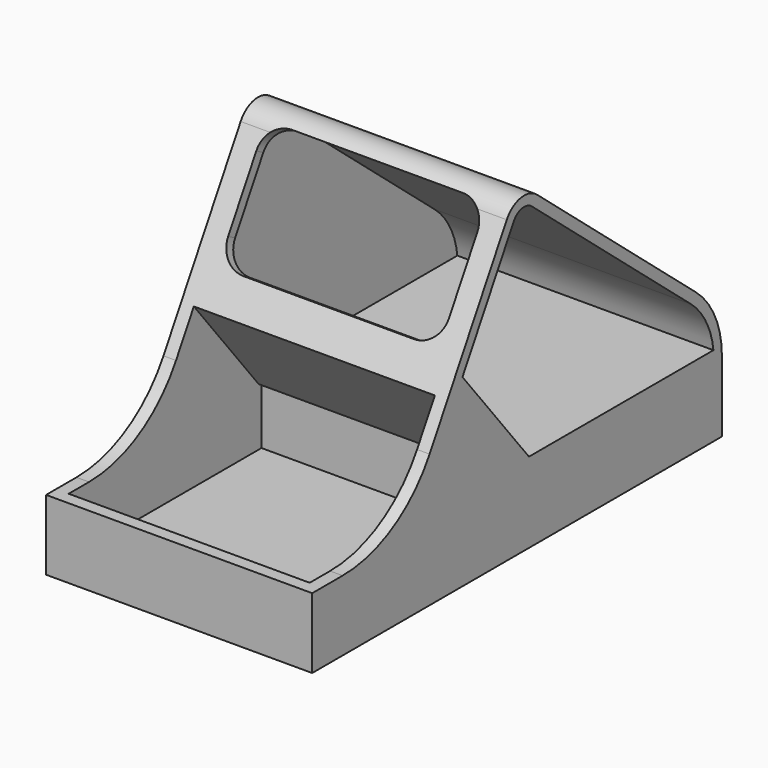
from build123d import *

# Parameters (mm, degrees)
F0_W      = 53
F0_H      = 53
F1_DEPTH  = 14
F0_H_2    = 49
F2_DEPTH  = 14
F3_T      = -2.5
F5_DEPTH  = 53
F6_DEPTH  = 53
F7_T      = -2.5
F9_R      = 18
F10_R     = 5
F11_T     = -2
F12_DEPTH = 7.2
F14_R     = 25


with BuildPart() as f1:
    # F0 (on Top) → F1 (new body)
    with BuildSketch(Plane.XY):
        with Locations((0, -24.5)):
            Rectangle(F0_W, F0_H)
    extrude(amount=F1_DEPTH)

    # F3
    f3_openings = [f1.faces().sort_by_distance(p)[0] for p in [
        (0, -24.5, 14),
    ]]
    offset(amount=F3_T, openings=f3_openings)


with BuildPart() as f2:
    # F0 (on Top) → F2 (new body)
    with BuildSketch(Plane.XY):
        with Locations((0, 26.5)):
            Rectangle(F0_W, F0_H_2)
    extrude(amount=F2_DEPTH)


with BuildPart() as f5:
    # F4 (on face) → F5 (new body, through all)
    with BuildSketch(Plane.YZ.offset(26.5)):
        Polygon((-16, 36.5), (2, 14), (51, 14), (51, 22.5), (0.4205387023, 64.94120732), align=None)
    extrude(amount=-F5_DEPTH)

    # F9
    f9_edges = [f5.edges().sort_by_distance(p)[0] for p in [
        (0, 51, 22.5),
    ]]
    fillet(f9_edges, radius=F9_R)

    # F10
    f10_edges = [f5.edges().sort_by_distance(p)[0] for p in [
        (0, 0.420539, 64.941207),
    ]]
    fillet(f10_edges, radius=F10_R)

    # F11
    f11_openings = [f5.faces().sort_by_distance(p)[0] for p in [
        (26.5, 14.357834, 32.967777),
    ]]
    offset(amount=F11_T, openings=f11_openings)

    # F8 (on face) → F12 (cut)
    with BuildSketch(Plane(origin=(0, -27.8049636191, 16.0532032303), x_dir=(1, 0, 0), z_dir=(0, -0.8660254038, 0.5))):
        with BuildLine():
            Line((17, 52.0304659404), (-17, 52.0304659404))
            ThreePointArc((-17, 52.0304659404), (-20.5355339059, 50.5659998464), (-22, 47.0304659404))
            Line((-22, 47.0304659404), (-22, 33.0304659404))
            ThreePointArc((-22, 33.0304659404), (-20.5355339059, 29.4949320345), (-17, 28.0304659404))
            Line((-17, 28.0304659404), (17, 28.0304659404))
            ThreePointArc((17, 28.0304659404), (20.5355339059, 29.4949320345), (22, 33.0304659404))
            Line((22, 33.0304659404), (22, 47.0304659404))
            ThreePointArc((22, 47.0304659404), (20.5355339059, 50.5659998464), (17, 52.0304659404))
        make_face()
    extrude(amount=-F12_DEPTH, mode=Mode.SUBTRACT)


with BuildPart() as f6:
    # F4 (on face) → F6 (new body, through all)
    with BuildSketch(Plane.YZ.offset(26.5)):
        Polygon((-16, 14), (2, 14), (-16, 36.5), align=None)
        Polygon((-16, 36.5), (-28.9903810568, 14), (-16, 14), align=None)
    extrude(amount=-F6_DEPTH)

    # F7
    f7_openings = [f6.faces().sort_by_distance(p)[0] for p in [
        (0, -22.495191, 25.25),
        (0, -13.495191, 14),
    ]]
    offset(amount=F7_T, openings=f7_openings)

    # F13: union F5, F2, F1
    add(f5.part)
    add(f2.part)
    add(f1.part)

    # F14
    f14_edges = [f6.edges().sort_by_distance(p)[0] for p in [
        (25.25, -28.990381, 14),
        (-25.25, -28.990381, 14),
    ]]
    fillet(f14_edges, radius=F14_R)


solid = f6.part
